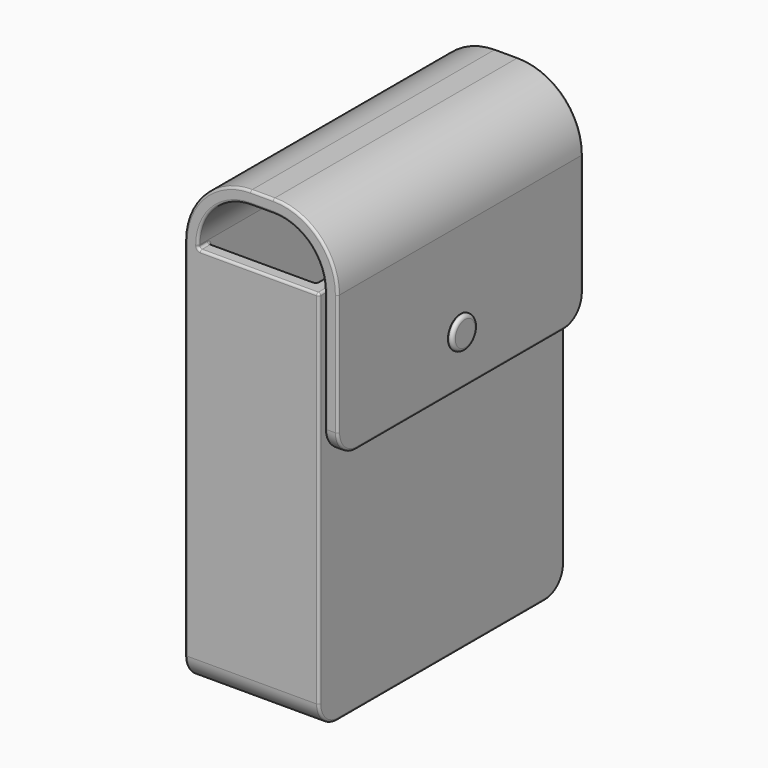
from build123d import *

# Parameters (mm, degrees)
F1_DEPTH = 32.8
F2_W     = 22.8530508727
F2_H     = 59.6
F3_DEPTH = 79.2
F4_R     = 5
F5_R     = 0.5
F6_R     = 3.3887140156
F7_DEPTH = 1.02
F8_R     = 0.7484062043
F9_R     = 0.0965685425


with BuildPart() as f1:
    # F0 (on Front) → F1 (new body, symmetric)
    with BuildSketch(Plane.XZ):
        with BuildLine():
            Line((-10.3166522458, 19.8068774239), (-10.3166522458, 19.1084556282))
            Line((-10.3166522458, 19.1084556282), (-7.5166523457, 19.1084556282))
            Line((-7.5166523457, 19.1084556282), (-7.5166523457, 19.8068774239))
            ThreePointArc((-7.5166523457, 19.8068774239), (-4.222440848, 27.759807499), (3.7304892271, 31.0540189967))
            Line((3.7304892271, 31.0540189967), (8.563811205, 31.0540189967))
            ThreePointArc((8.563811205, 31.0540189967), (16.3443622694, 27.831209223), (19.567172043, 20.0506581586))
            Line((19.567172043, 20.0506581586), (19.567172043, -10.8731621876))
            Line((19.567172043, -10.8731621876), (22.3671719432, -10.8731621876))
            Line((22.3671719432, -10.8731621876), (22.3671719432, 20.0506581586))
            ThreePointArc((22.3671719432, 20.0506581586), (18.3242611861, 29.8111081398), (8.563811205, 33.8540188968))
            Line((8.563811205, 33.8540188968), (3.7304892271, 33.8540188968))
            ThreePointArc((3.7304892271, 33.8540188968), (-6.2023397647, 29.7397064157), (-10.3166522458, 19.8068774239))
        make_face()
        Polygon((-7.5166523457, 19.1084556282), (-10.3166522458, 19.1084556282), (-10.3166522458, -63.2444918156), (18.336398527, -63.2444918156), (18.336398527, 19.1084556282), align=None)
    extrude(amount=F1_DEPTH, both=True)

    # F2 (on face) → F3 (cut)
    with BuildSketch(Plane.XY.offset(19.1084556282)):
        with Locations((3.9098730907, 0)):
            Rectangle(F2_W, F2_H)
    extrude(amount=-F3_DEPTH, mode=Mode.SUBTRACT)

    # F4
    f4_edges = [f1.edges().sort_by_distance(p)[0] for p in [
        (20.967172, -32.8, -10.873162),
        (20.967172, 32.8, -10.873162),
        (4.009873, 32.8, -63.244492),
        (4.009873, -32.8, -63.244492),
    ]]
    fillet(f4_edges, radius=F4_R)

    # F5
    f5_edges = [f1.edges().sort_by_distance(p)[0] for p in [
        (22.367172, -32.8, 7.088748),
        (6.14715, -32.8, 31.054019),
        (18.336399, -32.8, -19.568018),
        (5.409873, -32.8, 19.108456),
        (18.336399, 0, 19.108456),
        (3.909873, -29.8, 19.108456),
        (15.336399, 0, 19.108456),
        (15.336399, 29.8, -20.491544),
        (-7.516652, 29.8, -20.491544),
        (3.909873, 29.8, 19.108456),
        (3.909873, 29.8, -60.091544),
        (15.336399, -29.8, -20.491544),
        (15.336399, 0, -60.091544),
        (-7.516652, -29.8, -20.491544),
        (3.909873, -29.8, -60.091544),
        (-10.316652, 32.8, -19.218807),
        (-6.20234, 32.8, 29.739706),
        (18.336399, 32.8, -19.568018),
        (6.14715, 32.8, 33.854019),
        (5.409873, 32.8, 19.108456),
        (18.324261, 32.8, 29.811108),
        (22.367172, 32.8, 7.088748),
        (-4.222441, 32.8, 27.759807),
        (6.14715, 32.8, 31.054019),
        (19.567172, 32.8, 7.088748),
        (16.344362, 32.8, 27.831209),
        (-10.316652, 31.335534, -61.780026),
        (-10.316652, 0, -63.244492),
        (-10.316652, -32.8, -19.218807),
        (-10.316652, -31.335534, -61.780026),
        (18.336399, 31.335534, -61.780026),
        (-6.20234, -32.8, 29.739706),
        (18.336399, 0, -63.244492),
        (18.336399, -31.335534, -61.780026),
        (6.14715, -32.8, 33.854019),
        (-7.516652, -31.3, 19.108456),
        (-7.516652, 31.3, 19.108456),
        (18.324261, -32.8, 29.811108),
        (22.367172, 31.335534, -9.408696),
        (22.367172, 0, -10.873162),
        (22.367172, -31.335534, -9.408696),
        (-4.222441, -32.8, 27.759807),
        (19.567172, 31.335534, -9.408696),
        (19.567172, 0, -10.873162),
        (19.567172, -32.8, 7.088748),
        (19.567172, -31.335534, -9.408696),
        (16.344362, -32.8, 27.831209),
    ]]
    fillet(f5_edges, radius=F5_R)


with BuildPart() as f7:
    # F6 (on face) → F7 (new body)
    with BuildSketch(Plane.YZ.offset(22.3671719432)):
        Circle(F6_R)
    extrude(amount=F7_DEPTH)

    # F8
    f8_edges = [f7.edges().sort_by_distance(p)[0] for p in [
        (23.387172, -3.388714, 0),
    ]]
    fillet(f8_edges, radius=F8_R)

    # F9
    f9_edges = [f7.edges().sort_by_distance(p)[0] for p in [
        (22.367172, -3.388714, 0),
    ]]
    fillet(f9_edges, radius=F9_R)


solid = Compound([f1.part, f7.part])
